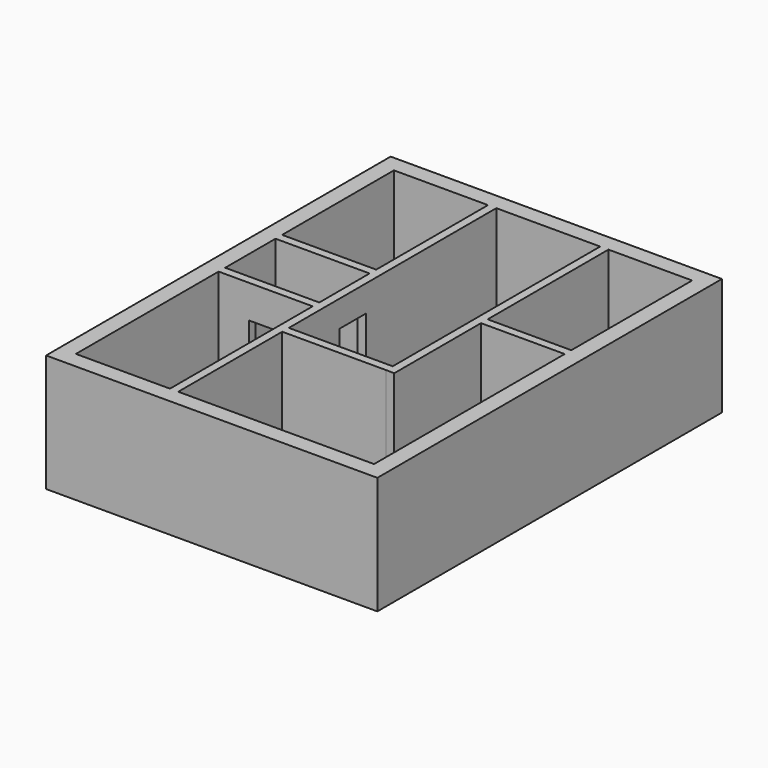
from build123d import *

# Parameters (mm, degrees)
F0_W     = 10000
F0_H     = 13000
F1_DEPTH = 3550
F2_W     = 9000
F2_H     = 12000
F3_DEPTH = 3300
F5_DEPTH = 3300
F6_W     = 1000
F6_H     = 2300
F7_DEPTH = 250
F8_W     = 1000
F8_H     = 2500
F9_DEPTH = 250


# Not quite as in the source:
# - a feature names something its author has since deleted; it is built from what else it names


with BuildPart() as f1:
    # F0 (on Top) → F1 (new body)
    with BuildSketch(Plane.XY):
        Rectangle(F0_W, F0_H)
    extrude(amount=F1_DEPTH)

    # F2 (on face) → F3 (cut)
    with BuildSketch(Plane.XY.offset(3550)):
        Rectangle(F2_W, F2_H)
    extrude(amount=-F3_DEPTH, mode=Mode.SUBTRACT)

    # F4 (on face) → F5 (join)
    with BuildSketch(Plane.XY.offset(250)):
        Polygon((-1660.4968309402, -366.6217029095), (-4500, -366.6217029095), (-4500, -616.6217029095), (-1660.4968309402, -616.6217029095), (-1660.4968309402, -6000), (-1410.4968309402, -6000), (-1410.4968309402, -2077.5351682588), (1725.1923292822, -2077.5351682588), (1975.1266148544, -2083.2669128011), (1975.1876689086, 1191.9026374817), (4500, 1191.9026374817), (4500, 1441.9026374817), (1975.1923292822, 1441.9026374817), (1975.1923292822, 6000), (1725.1923292822, 6000), (1725.1923292822, 1441.9026374817), (1725.1923292822, -1827.5351682588), (-1410.4968309402, -1827.5351682588), (-1410.4968309402, 6000), (-1660.4968309402, 6000), (-1660.4968309402, 1781.4515829086), (-4500, 1781.4515829086), (-4500, 1531.4515829086), (-1660.4968309402, 1531.4515829086), align=None)
    extrude(amount=F5_DEPTH)

    # F6 (on face) → F7 (cut)
    with BuildSketch(Plane.XZ.offset(616.6217029095)):
        with Locations((-3080.2484154701, 1400)):
            Rectangle(F6_W, F6_H)
    extrude(amount=-F7_DEPTH, mode=Mode.SUBTRACT)

    # F8 (on face) → F9 (cut, through all)
    with BuildSketch(Plane(origin=(-1660.4968309402, 0, 0), x_dir=(0, -1, 0), z_dir=(-1, 0, 0))):
        with Locations((-582.4149399996, 1500)):
            Rectangle(F8_W, F8_H)
    extrude(amount=-F9_DEPTH, mode=Mode.SUBTRACT)


solid = f1.part
